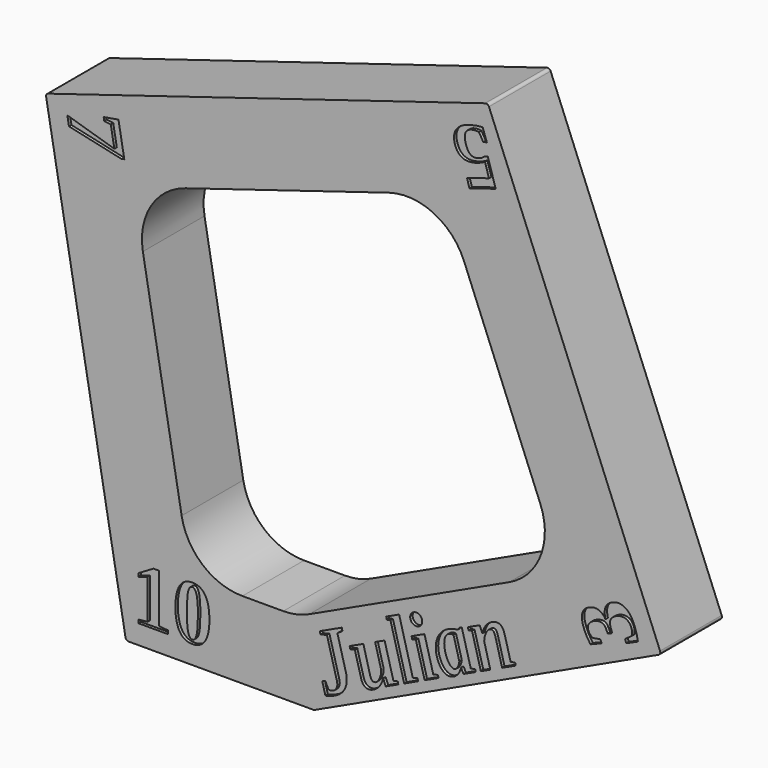
from build123d import *

# Parameters (mm, degrees)
F1_DEPTH     = 6.35
F3_DEPTH     = 6.351
F4_R         = 0.254
F5_TEXT_SIZE = 6.6145833333
F6_DEPTH     = 0.254


# Not quite as in the source:
# - Text() gives the source's letters only with a copy of the font that has no kerning and outlines rounded to 1/6400 em; it was checked with that copy


with BuildPart() as f1:
    # F0 (on Front) → F1 (new body)
    with BuildSketch(Plane.XZ):
        Polygon((12.3523935342, 25.8973315975), (-24.082817668, 14.7579696476), (-17.4668220989, -22.7632057422), (-1.9717357954, -22.7632057422), (26.6249047433, -9.4283732615), align=None)
    extrude(amount=F1_DEPTH)

    # F2 (on face) → F3 (cut, through all)
    with BuildSketch(Plane.XZ.offset(6.35)):
        with BuildLine():
            ThreePointArc((-12.555711782, 11.6420169317), (-15.4018755569, 9.4382814801), (-16.0732869073, 5.9018560288))
            Line((-16.0732869073, 5.9018560288), (-12.8787366998, -12.2153384847))
            ThreePointArc((-12.8787366998, -12.2153384847), (-11.1412743717, -15.2247115132), (-7.8759133145, -16.4132057422))
            Line((-7.8759133145, -16.4132057422), (-4.5057057894, -16.4132057422))
            ThreePointArc((-4.5057057894, -16.4132057422), (-3.4061925506, -16.2927894584), (-2.3588050197, -15.9372493003))
            Line((-2.3588050197, -15.9372493003), (14.1108618306, -8.2573175207))
            ThreePointArc((14.1108618306, -8.2573175207), (16.6904823063, -5.5151001944), (16.6740550422, -1.750272468))
            Line((16.6740550422, -1.750272468), (10.3882801434, 13.8075663474))
            ThreePointArc((10.3882801434, 13.8075663474), (7.865182534, 16.4896980973), (4.1929379022, 16.7625930131))
            Line((4.1929379022, 16.7625930131), (-12.555711782, 11.6420169317))
        make_face()
    extrude(amount=-F3_DEPTH, mode=Mode.SUBTRACT)

    # F4
    f4_edges = [f1.edges().sort_by_distance(p)[0] for p in [
        (-24.082818, -3.175, 14.75797),
        (12.352394, -3.175, 25.897332),
        (26.624905, -3.175, -9.428373),
        (-1.971736, -3.175, -22.763206),
        (-17.466822, -3.175, -22.763206),
    ]]
    fillet(f4_edges, radius=F4_R)

    # F5 (on face) → F6 (cut)
    with BuildSketch(Plane.XZ.offset(6.35)):
        with Locations((-16.9529911808, -21.1757057422)):
            Text('10', F5_TEXT_SIZE, font='Tinos', font_style=FontStyle.BOLD, text_align=(TextAlign.LEFT, TextAlign.BOTTOM))
        with Locations(Location((-22.415449707, 14.4439041859), (0, 0, -80))):
            Text('7', F5_TEXT_SIZE, font='Tinos', font_style=FontStyle.BOLD, text_align=(TextAlign.LEFT, TextAlign.BOTTOM))
        with Locations(Location((12.1902862126, 24.1877347522), (0, 0, -163))):
            Text('5', F5_TEXT_SIZE, font='Tinos', font_style=FontStyle.BOLD, text_align=(TextAlign.LEFT, TextAlign.BOTTOM))
        with Locations(Location((24.8868226664, -9.3642482833), (0, 0, 112))):
            Text('3', F5_TEXT_SIZE, font='Tinos', font_style=FontStyle.BOLD, text_align=(TextAlign.LEFT, TextAlign.BOTTOM))
        with Locations(Location((-1.0101486085, -21.4390040498), (0, 0, 25))):
            Text('Julian', F5_TEXT_SIZE, font='Tinos', font_style=FontStyle.BOLDITALIC, text_align=(TextAlign.LEFT, TextAlign.BOTTOM))
    extrude(amount=-F6_DEPTH, mode=Mode.SUBTRACT)


solid = f1.part
